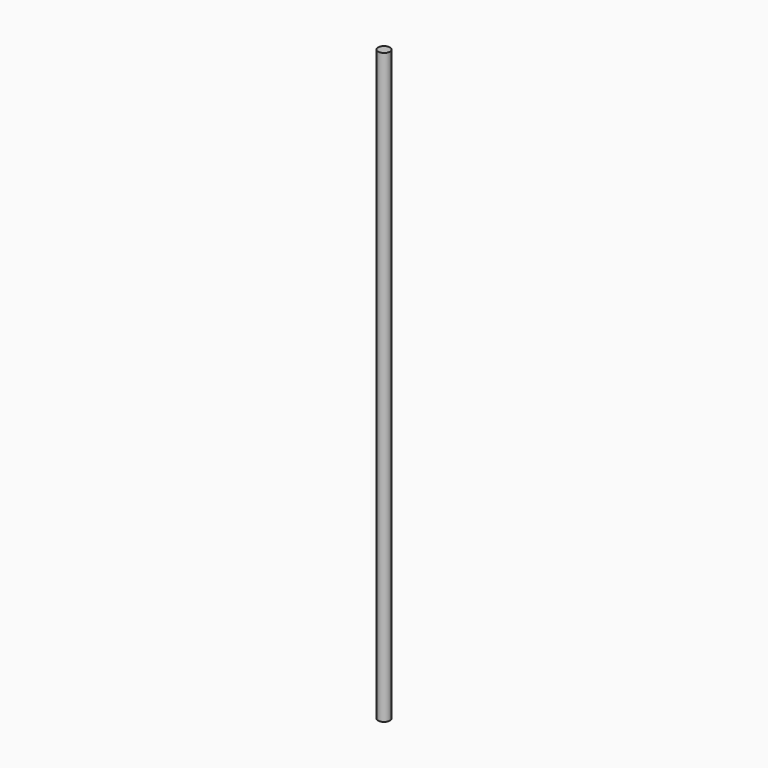
from build123d import *

# Parameters (mm, degrees)
F0_R     = 19.05
F3_DEPTH = 1917.7


# Not quite as in the source:
# - the program builds the solid bodies; features that only make, move or delete a surface that nothing else refers to are left out


with BuildPart() as f3:
    # F0 (on Top) → F3 (new body)
    with BuildSketch(Plane.XY):
        with Locations((0, 895.35)):
            Circle(F0_R)
    extrude(amount=F3_DEPTH)


solid = f3.part
